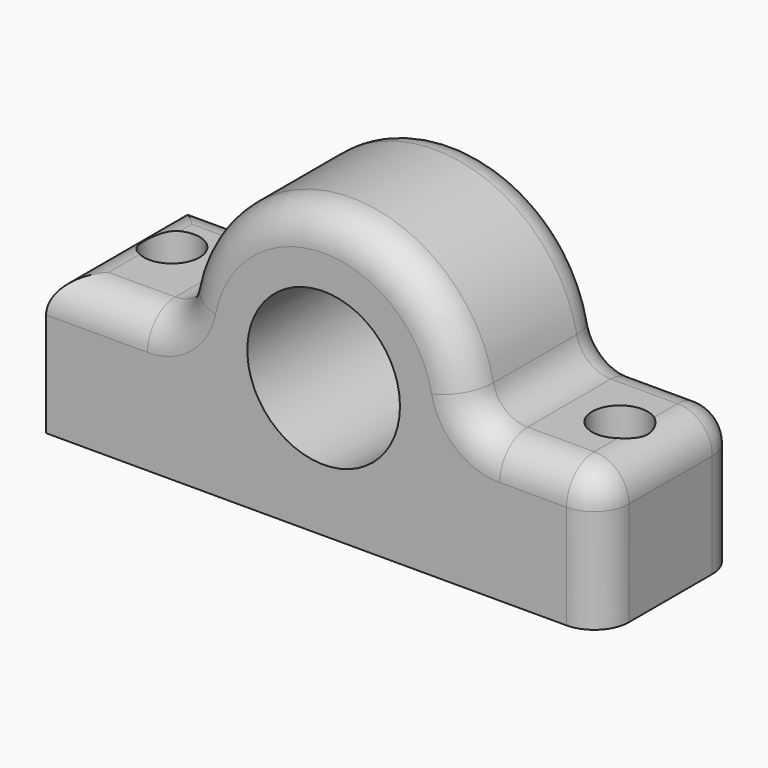
from build123d import *

# Parameters (mm, degrees)
F0_R         = 11
F1_DEPTH     = 25
F2_R         = 4
F4_DEPTH     = 25
F3_R         = 4
F5_DEPTH     = 25
F6_S2_W      = 5
F6_S2_H      = 5
F6_T3_DEPTH  = 5
F6_T8_ANGLE  = 157.7136601513
F6_T11_DEPTH = 32.5
F6_T14_DEPTH = 27.5
F6_T17_ANGLE = 157.7136601513
F6_T20_DEPTH = 50
F6_T23_ANGLE = 78.8568300757
F6_T26_ANGLE = 78.8568300757
F6_T29_DEPTH = 27.1160389937
F6_T32_DEPTH = 27.1160389937
F6_T35_ANGLE = 78.8568300757
F6_T38_ANGLE = 78.8568300757
F6_T41_DEPTH = 27.1160389937
F6_T44_DEPTH = 9.6160389937
F7_T1_DEPTH  = 27.5
F7_S5_W      = 5
F7_S5_H      = 5
F7_T6_DEPTH  = 5


# Not quite as in the source:
# - a fillet or chamfer that OpenCascade refuses, or shapes differently, is made with other operations: its cross-section is extruded or revolved along the edge and cut away or added


with BuildPart() as f1:
    # F0 (on Front) → F1 (new body)
    with BuildSketch(Plane.XZ):
        with BuildLine():
            Line((-40, 10), (-40, -10))
            Line((-40, -10), (40, -10))
            Line((40, -10), (40, 10))
            Line((40, 10), (25.3839610063, 10))
            ThreePointArc((25.3839610063, 10), (22.2083926988, 11.137906536), (20.4782243644, 14.0336936303))
            ThreePointArc((20.4782243644, 14.0336936303), (0, 30.8717118949), (-20.4782243644, 14.0336936303))
            ThreePointArc((-20.4782243644, 14.0336936303), (-22.2083926988, 11.137906536), (-25.3839610063, 10))
            Line((-25.3839610063, 10), (-40, 10))
        make_face()
        with Locations((0, 10)):
            Circle(F0_R, mode=Mode.SUBTRACT)
    extrude(amount=F1_DEPTH)

    # F2 (on face) → F4 (cut)
    with BuildSketch(Plane.XY.offset(10)):
        with Locations((32.6919805032, -12.5)):
            Circle(F2_R)
    extrude(amount=-F4_DEPTH, mode=Mode.SUBTRACT)

    # F3 (on face) → F5 (cut)
    with BuildSketch(Plane.XY.offset(10)):
        with Locations((-33.267121762, -10.7605047524)):
            Circle(F3_R)
    extrude(amount=-F5_DEPTH, mode=Mode.SUBTRACT)

    # F6: fillet of radius 5 on 5 edges, made by hand


with BuildPart() as f6_tool1:
    # F6_s2 → F6_t3 (new body)
    with BuildSketch(Plane.YZ.offset(35)):
        with Locations((-22.5, 7.5)):
            Rectangle(F6_S2_W, F6_S2_H)
    extrude(amount=F6_T3_DEPTH)

    # F6_s4 → F6_t5 (revolve, cut)
    with BuildSketch(Plane(origin=(35, -20, 5), x_dir=(0, 0.7071067812, -0.7071067812), z_dir=(0, -0.7071067812, -0.7071067812))):
        with BuildLine():
            ThreePointArc((0, -5), (5, 0), (0, 5))
            Line((0, 5), (0, -5))
        make_face()
    revolve(axis=Axis((35, -20, 5), (1, 0, 0)), mode=Mode.SUBTRACT)


with BuildPart() as f6_tool6:
    # F6_s7 → F6_t8 (revolve)
    with BuildSketch(Plane(origin=(-1.8961778261, 0, 9.6265007999), x_dir=(0, 1, 0), z_dir=(0.1932612739, 0, -0.9811473284))):
        with BuildLine():
            ThreePointArc((-20, 22.8043246343), (-23.5355339059, 21.3398585403), (-25, 17.8043246343))
            Line((-25, 17.8043246343), (-25, 22.8043246343))
            Line((-25, 22.8043246343), (-20, 22.8043246343))
        make_face()
    revolve(axis=Axis((0, -25, 10), (0, -1, 0)), revolution_arc=F6_T8_ANGLE)


with BuildPart() as f6_tool9:
    # F6_s10 → F6_t11 (new body)
    with BuildSketch(Plane.XZ.offset(-12.5)):
        with BuildLine():
            ThreePointArc((40, 5), (38.5355339059, 8.5355339059), (35, 10))
            Line((35, 10), (40, 10))
            Line((40, 10), (40, 5))
        make_face()
    extrude(amount=F6_T11_DEPTH)


with BuildPart() as f6_tool12:
    # F6_s13 → F6_t14 (new body)
    with BuildSketch(Plane.XY.offset(-22.5)):
        with BuildLine():
            ThreePointArc((35, -25), (38.5355339059, -23.5355339059), (40, -20))
            Line((40, -20), (40, -25))
            Line((40, -25), (35, -25))
        make_face()
    extrude(amount=F6_T14_DEPTH)


with BuildPart() as f6_tool15:
    # F6_s16 → F6_t17 (revolve)
    with BuildSketch(Plane(origin=(-1.8961778261, 0, 9.6265007999), x_dir=(0, 1, 0), z_dir=(0.1932612739, 0, -0.9811473284))):
        with BuildLine():
            ThreePointArc((-5, 22.8043246343), (-1.4644660941, 21.3398585403), (0, 17.8043246343))
            Line((0, 17.8043246343), (0, 22.8043246343))
            Line((0, 22.8043246343), (-5, 22.8043246343))
        make_face()
    revolve(axis=Axis((0, 0, 10), (0, -1, 0)), revolution_arc=F6_T17_ANGLE)


with BuildPart() as f6_tool18:
    # F6_s19 → F6_t20 (new body)
    with BuildSketch(Plane.XZ.offset(-12.5)):
        with BuildLine():
            ThreePointArc((-35, 10), (-38.5355339059, 8.5355339059), (-40, 5))
            Line((-40, 5), (-40, 10))
            Line((-40, 10), (-35, 10))
        make_face()
    extrude(amount=F6_T20_DEPTH)


with BuildPart() as f6_tool21:
    # F6_s22 → F6_t23 (revolve)
    with BuildSketch(Plane.YZ.offset(25.3839610063)):
        with BuildLine():
            ThreePointArc((0, 5), (-1.4644660941, 8.5355339059), (-5, 10))
            Line((-5, 10), (0, 10))
            Line((0, 10), (0, 5))
        make_face()
    revolve(axis=Axis((25.3839610063, 0, 15), (0, 1, 0)), revolution_arc=F6_T23_ANGLE)


with BuildPart() as f6_tool24:
    # F6_s25 → F6_t26 (revolve)
    with BuildSketch(Plane(origin=(1.8961778261, 0, 9.6265007999), x_dir=(0, 1, 0), z_dir=(0.1932612739, 0, 0.9811473284))):
        with BuildLine():
            ThreePointArc((-5, 22.8043246343), (-1.4644660941, 21.3398585403), (0, 17.8043246343))
            Line((0, 17.8043246343), (0, 22.8043246343))
            Line((0, 22.8043246343), (-5, 22.8043246343))
        make_face()
    revolve(axis=Axis((-25.3839610063, 0, 15), (0, 1, 0)), revolution_arc=F6_T26_ANGLE)


with BuildPart() as f6_tool27:
    # F6_s28 → F6_t29 (new body)
    with BuildSketch(Plane.YZ.offset(-25.3839610063)):
        with BuildLine():
            ThreePointArc((-5, 10), (-1.4644660941, 8.5355339059), (0, 5))
            Line((0, 5), (0, 10))
            Line((0, 10), (-5, 10))
        make_face()
    extrude(amount=-F6_T29_DEPTH)


with BuildPart() as f6_tool30:
    # F6_s31 → F6_t32 (new body)
    with BuildSketch(Plane.YZ.offset(52.5)):
        with BuildLine():
            ThreePointArc((0, 5), (-1.4644660941, 8.5355339059), (-5, 10))
            Line((-5, 10), (0, 10))
            Line((0, 10), (0, 5))
        make_face()
    extrude(amount=-F6_T32_DEPTH)


with BuildPart() as f6_tool33:
    # F6_s34 → F6_t35 (revolve)
    with BuildSketch(Plane.YZ.offset(25.3839610063)):
        with BuildLine():
            ThreePointArc((-25, 5), (-23.5355339059, 8.5355339059), (-20, 10))
            Line((-20, 10), (-25, 10))
            Line((-25, 10), (-25, 5))
        make_face()
    revolve(axis=Axis((25.3839610063, -25, 15), (0, 1, 0)), revolution_arc=F6_T35_ANGLE)


with BuildPart() as f6_tool36:
    # F6_s37 → F6_t38 (revolve)
    with BuildSketch(Plane(origin=(1.8961778261, 0, 9.6265007999), x_dir=(0, 1, 0), z_dir=(0.1932612739, 0, 0.9811473284))):
        with BuildLine():
            ThreePointArc((-20, 22.8043246343), (-23.5355339059, 21.3398585403), (-25, 17.8043246343))
            Line((-25, 17.8043246343), (-25, 22.8043246343))
            Line((-25, 22.8043246343), (-20, 22.8043246343))
        make_face()
    revolve(axis=Axis((-25.3839610063, -25, 15), (0, 1, 0)), revolution_arc=F6_T38_ANGLE)


with BuildPart() as f6_tool39:
    # F6_s40 → F6_t41 (new body)
    with BuildSketch(Plane.YZ.offset(-25.3839610063)):
        with BuildLine():
            ThreePointArc((-20, 10), (-23.5355339059, 8.5355339059), (-25, 5))
            Line((-25, 5), (-25, 10))
            Line((-25, 10), (-20, 10))
        make_face()
    extrude(amount=-F6_T41_DEPTH)


with BuildPart() as f6_tool42:
    # F6_s43 → F6_t44 (new body)
    with BuildSketch(Plane.YZ.offset(35)):
        with BuildLine():
            ThreePointArc((-25, 5), (-23.5355339059, 8.5355339059), (-20, 10))
            Line((-20, 10), (-25, 10))
            Line((-25, 10), (-25, 5))
        make_face()
    extrude(amount=-F6_T44_DEPTH)


with BuildPart() as f1_1:
    add(f1.part)

    # F6_t45: cut F6_tool1, F6_tool6, F6_tool9, F6_tool12, F6_tool15, F6_tool18, F6_tool21, F6_tool24, F6_tool27, F6_tool30, F6_tool33, F6_tool36, F6_tool39, F6_tool42
    add([f6_tool1.part, f6_tool6.part, f6_tool9.part, f6_tool12.part, f6_tool15.part, f6_tool18.part, f6_tool21.part, f6_tool24.part, f6_tool27.part, f6_tool30.part, f6_tool33.part, f6_tool36.part, f6_tool39.part, f6_tool42.part], mode=Mode.SUBTRACT)

    # F7: fillet of radius 5 on 1 edges, made by hand

    # F7_s2 → F7_t1 (cut)
    with BuildSketch(Plane.XY.offset(-22.5)):
        with BuildLine():
            ThreePointArc((35, 0), (38.5355339059, -1.4644660941), (40, -5))
            Line((40, -5), (40, 0))
            Line((40, 0), (35, 0))
        make_face()
    extrude(amount=F7_T1_DEPTH, mode=Mode.SUBTRACT)


with BuildPart() as f7_tool4:
    # F7_s5 → F7_t6 (new body)
    with BuildSketch(Plane.XZ.offset(5)):
        with Locations((37.5, 7.5)):
            Rectangle(F7_S5_W, F7_S5_H)
    extrude(amount=-F7_T6_DEPTH)

    # F7_s7 → F7_t8 (revolve, cut)
    with BuildSketch(Plane(origin=(35, -5, 5), x_dir=(-0.7071067812, 0, -0.7071067812), z_dir=(0.7071067812, 0, -0.7071067812))):
        with BuildLine():
            ThreePointArc((0, -5), (5, 0), (0, 5))
            Line((0, 5), (0, -5))
        make_face()
    revolve(axis=Axis((35, -5, 5), (0, 1, 0)), mode=Mode.SUBTRACT)


with BuildPart() as f1_2:
    add(f1_1.part)

    # F7_t3: cut F7_tool4
    add(f7_tool4.part, mode=Mode.SUBTRACT)


solid = f1_2.part
